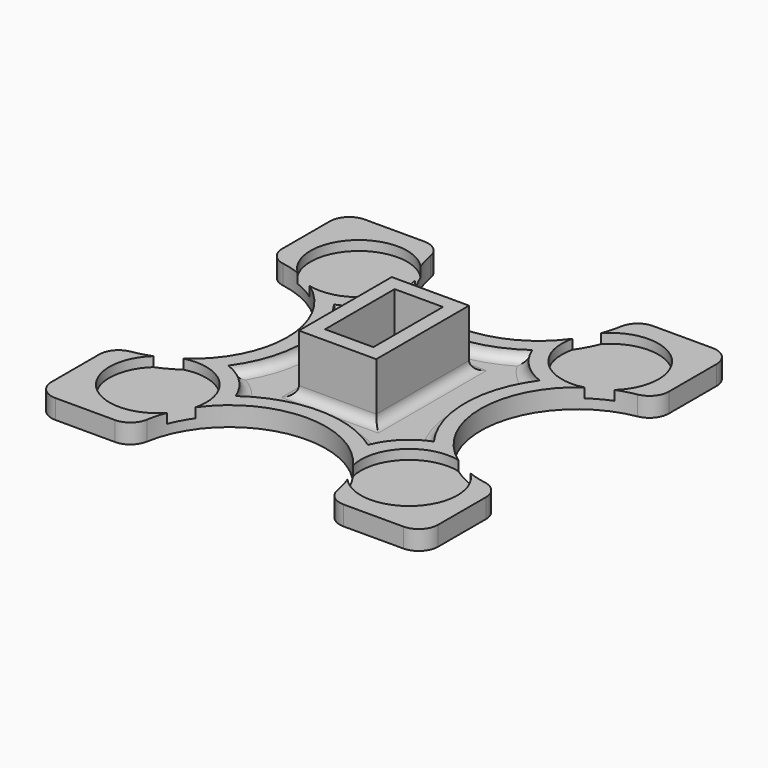
from build123d import *

# Parameters (mm, degrees)
F0_W      = 101.6
F0_H      = 101.6
F1_DEPTH  = 5.08
F2_R      = 12.7
F3_DEPTH  = 2.54
F4_W      = 20.32
F4_H      = 30.48
F4_W_2    = 12.7
F4_H_2    = 22.86
F5_DEPTH  = 12.7
F6_R      = 25.4
F7_DEPTH  = 25.4
F8_R      = 5.08
F9_W      = 20.32
F9_H      = 30.48
F10_DEPTH = 2.54
F11_R     = 2.53999


# Not quite as in the source:
# - a fillet or chamfer is up to 0.001 mm smaller than in the source, because OpenCascade refuses the exact size


with BuildPart() as f1:
    # F0 (on Top) → F1 (new body)
    with BuildSketch(Plane.XY):
        Rectangle(F0_W, F0_H)
    extrude(amount=F1_DEPTH)

    # F2 (on face) → F3 (cut)
    with BuildSketch(Plane.XY.offset(5.08)):
        with Locations((-33.02, 33.02)):
            Circle(F2_R)
        with Locations((33.02, 33.02)):
            Circle(F2_R)
        with Locations((33.02, -33.02)):
            Circle(F2_R)
        with Locations((-33.02, -33.02)):
            Circle(F2_R)
    extrude(amount=-F3_DEPTH, mode=Mode.SUBTRACT)

    # F4 (on face) → F5 (join)
    with BuildSketch(Plane.XY.offset(5.08)):
        Rectangle(F4_W, F4_H)
        Rectangle(F4_W_2, F4_H_2, mode=Mode.SUBTRACT)
    extrude(amount=F5_DEPTH)

    # F6 (on face) → F7 (cut)
    with BuildSketch(Plane.XY.offset(5.08)):
        with Locations((-50.8, 0)):
            Circle(F6_R)
        with Locations((50.8, 0)):
            Circle(F6_R)
        with Locations((0, 50.8)):
            Circle(F6_R)
        with Locations((0, -50.8)):
            Circle(F6_R)
    extrude(amount=-F7_DEPTH, mode=Mode.SUBTRACT)

    # F8
    f8_edges = [f1.edges().sort_by_distance(p)[0] for p in [
        (-50.8, -25.4, 2.54),
        (-50.8, 25.4, 2.54),
        (-50.8, -50.8, 2.54),
        (25.4, -50.8, 2.54),
        (-25.4, -50.8, 2.54),
        (50.8, -50.8, 2.54),
        (50.8, -25.4, 2.54),
        (50.8, 25.4, 2.54),
        (50.8, 50.8, 2.54),
        (-25.4, 50.8, 2.54),
        (25.4, 50.8, 2.54),
        (-50.8, 50.8, 2.54),
    ]]
    fillet(f8_edges, radius=F8_R)

    # F9 (on face) → F10 (cut)
    with BuildSketch(Plane.XY.offset(5.08)):
        with BuildLine():
            ThreePointArc((27.0028755866, -17.3730866956), (21.3360004127, 0), (27.0028755866, 17.3730866956))
            ThreePointArc((27.0028755866, 17.3730866956), (21.166062212, 21.166062212), (17.3730866956, 27.0028755866))
            ThreePointArc((17.3730866956, 27.0028755866), (0, 21.3360004127), (-17.3730866956, 27.0028755866))
            ThreePointArc((-17.3730866956, 27.0028755866), (-21.166062212, 21.166062212), (-27.0028755866, 17.3730866956))
            ThreePointArc((-27.0028755866, 17.3730866956), (-21.3360004127, 0), (-27.0028755866, -17.3730866956))
            ThreePointArc((-27.0028755866, -17.3730866956), (-21.166062212, -21.166062212), (-17.3730866956, -27.0028755866))
            ThreePointArc((-17.3730866956, -27.0028755866), (0, -21.3360004127), (17.3730866956, -27.0028755866))
            ThreePointArc((17.3730866956, -27.0028755866), (21.166062212, -21.166062212), (27.0028755866, -17.3730866956))
        make_face()
        Rectangle(F9_W, F9_H, mode=Mode.SUBTRACT)
    extrude(amount=-F10_DEPTH, mode=Mode.SUBTRACT)

    # F11 (radius 2.54 in the source; OpenCascade refuses exactly that, so slightly less here)
    f11_edges = [f1.edges().sort_by_distance(p)[0] for p in [
        (21.336, 0, 2.54),
        (21.166062, 21.166062, 2.54),
        (0, 21.336, 2.54),
        (-21.166062, 21.166062, 2.54),
        (-21.336, 0, 2.54),
        (-21.166062, -21.166062, 2.54),
        (0, -21.336, 2.54),
        (21.166062, -21.166062, 2.54),
        (-10.16, 0, 2.54),
        (0, 15.24, 2.54),
        (10.16, 0, 2.54),
        (0, -15.24, 2.54),
    ]]
    fillet(f11_edges, radius=F11_R)


solid = f1.part
